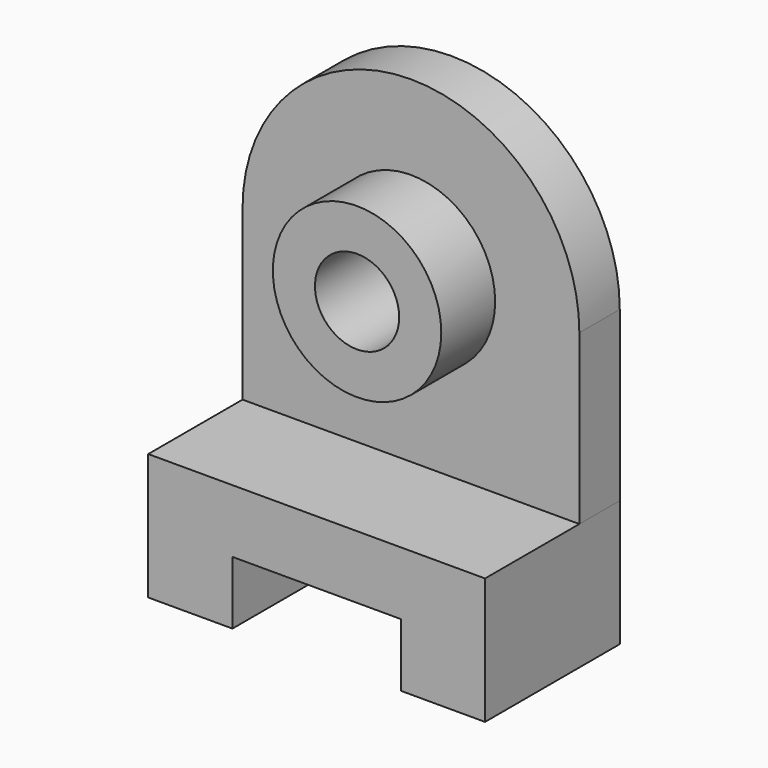
from build123d import *

# Parameters (mm, degrees)
F0_R     = 20
F0_R_2   = 10
F1_DEPTH = 28
F2_DEPTH = 12
F3_DEPTH = 40


# Not quite as in the source:
# - ends of sketch curves that miss each other by under 0.0002 mm in the source are joined


with BuildPart() as f1:
    # F0 (on Front) → F1 (new body)
    with BuildSketch(Plane.XZ):
        with Locations((0, 36.7759418548)):
            Circle(F0_R)
        with Locations((0, 36.7759418548)):
            Circle(F0_R_2, mode=Mode.SUBTRACT)
    extrude(amount=F1_DEPTH)

    # F0 (on Front) → F2 (join)
    with BuildSketch(Plane.XZ):
        with BuildLine():
            ThreePointArc((40, 36.7759418548), (0, 76.7759418548), (-40, 36.7759418548))
            Line((-40, 36.7759418548), (-40.0000252162, -3.2240581452))
            Line((-40.0000252162, -3.2240581452), (39.9999747838, -3.2240581452))
            Line((39.9999747838, -3.2240581452), (40, 36.7759418548))
        make_face()
        with Locations((0, 36.7759418548)):
            Circle(F0_R, mode=Mode.SUBTRACT)
    extrude(amount=F2_DEPTH)

    # F0 (on Front) → F3 (join)
    with BuildSketch(Plane.XZ):
        Polygon((39.9999747838, -3.2240581452), (-40, -3.2240581452), (-40.0000441283, -33.2240581452), (-20.0000441283, -33.2240707533), (-20.0000346722, -18.2240707533), (19.9999653278, -18.2240623479), (19.9999558717, -33.2240623479), (39.9999558717, -33.2240581452), align=None)
    extrude(amount=F3_DEPTH)


solid = f1.part
